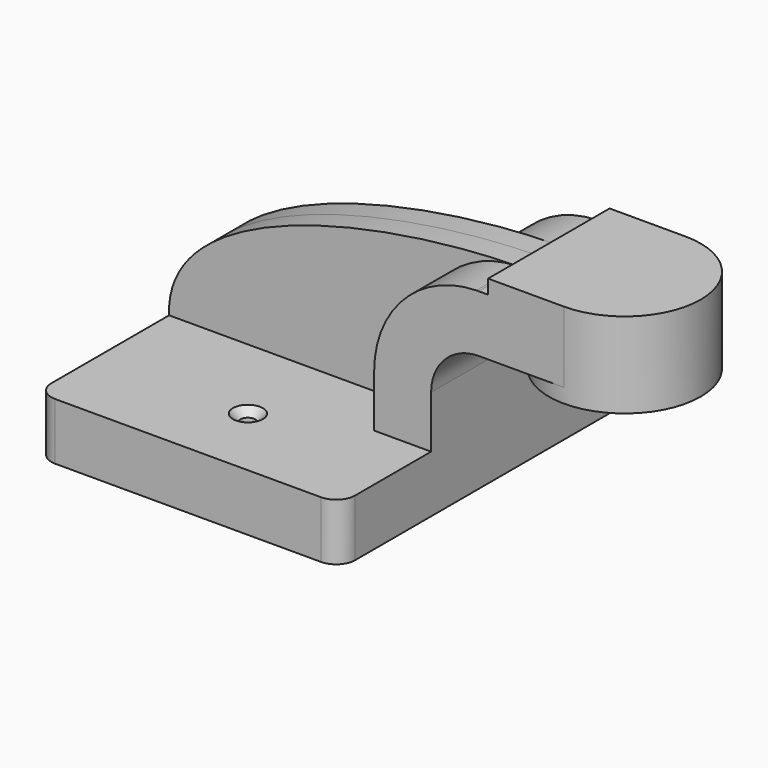
from build123d import *

# Parameters (mm, degrees)
F1_DEPTH       = 63.5
F2_DEPTH       = 25.4
F3_DEPTH       = 7.9375
F5_R           = 6.35
F7_D           = 5
F7_CSINK_D     = 10
F7_CSINK_ANGLE = 90


# Not quite as in the source:
# - a feature names something its author has since deleted; it is built from what else it names


with BuildPart() as f1:
    # F0 (on Front) → F1 (new body, symmetric)
    with BuildSketch(Plane.XZ):
        Polygon((31.75, 9.525), (-50.8, 9.525), (-50.8, -9.525), (50.8, -9.525), (50.8, 9.525), align=None)
    extrude(amount=F1_DEPTH, both=True)

    # F0 (on Front) → F2 (join, symmetric)
    with BuildSketch(Plane.XZ):
        with BuildLine():
            Line((31.75, 27.0002), (31.75, 9.525))
            Line((31.75, 9.525), (50.8, 9.525))
            Line((50.8, 9.525), (50.8, 27.0002))
            ThreePointArc((50.8, 27.0002), (55.4496798487, 38.2255201513), (66.675, 42.8752))
            Line((66.675, 42.8752), (69.85, 42.8752))
            Line((69.85, 42.8752), (69.85, 61.9252))
            Line((69.85, 61.9252), (66.675, 61.9252))
            add(Edge.make_bspline(
                [(65.9455207974, 61.9175808453), (66.1893918553, 61.9205374951), (66.4325563897, 61.9230769491), (66.675, 61.9252)],
                knots=[127.9589342237, 127.9589342237, 127.9589342237, 127.9589342237, 128.6318645789, 128.6318645789, 128.6318645789, 128.6318645789], degree=3))
            ThreePointArc((65.9455207974, 61.9175808453), (41.72271868, 51.4366334944), (31.75, 27.0002))
        make_face()
        Polygon((69.85, 66.675), (69.85, 61.9252), (69.85, 42.8752), (95.25, 42.8752), (95.25, 66.675), align=None)
    extrude(amount=F2_DEPTH, both=True)

    # F0 (on Front) → F3 (join, symmetric)
    with BuildSketch(Plane.XZ):
        with BuildLine():
            add(Edge.make_bspline(
                [(-50.8, 9.525), (-52.3458055459, 45.7083043223), (19.5729944142, 61.3553684788), (65.9455207974, 61.9175808453)],
                knots=[0, 0, 0, 0, 127.9589342237, 127.9589342237, 127.9589342237, 127.9589342237], degree=3))
            Line((-50.8, 9.525), (31.75, 9.525))
            Line((31.75, 9.525), (31.75, 27.0002))
            ThreePointArc((31.75, 27.0002), (41.72271868, 51.4366334944), (65.9455207974, 61.9175808453))
        make_face()
    extrude(amount=F3_DEPTH, both=True)

    # F0 (on Front) → F4 (revolve)
    with BuildSketch(Plane.XZ):
        Polygon((120.65, 66.675), (95.25, 66.675), (95.25, 42.8752), (95.25, 38.1), (120.65, 38.1), align=None)
    revolve(axis=Axis((95.25, 0, 52.3875), (0, 0, 1)))

    # F5
    f5_edges = [f1.edges().sort_by_distance(p)[0] for p in [
        (50.8, -63.5, 0),
        (-50.8, -63.5, 0),
        (-50.8, 63.5, 0),
        (50.8, 63.5, 0),
    ]]
    fillet(f5_edges, radius=F5_R)

    # F7 (through all)
    with Locations(Plane.XY.offset(9.525)):
        with Locations((0, 36.2676680088), (0, -38.4938158095)):
            CounterSinkHole(F7_D / 2, F7_CSINK_D / 2, counter_sink_angle=F7_CSINK_ANGLE)


solid = f1.part
